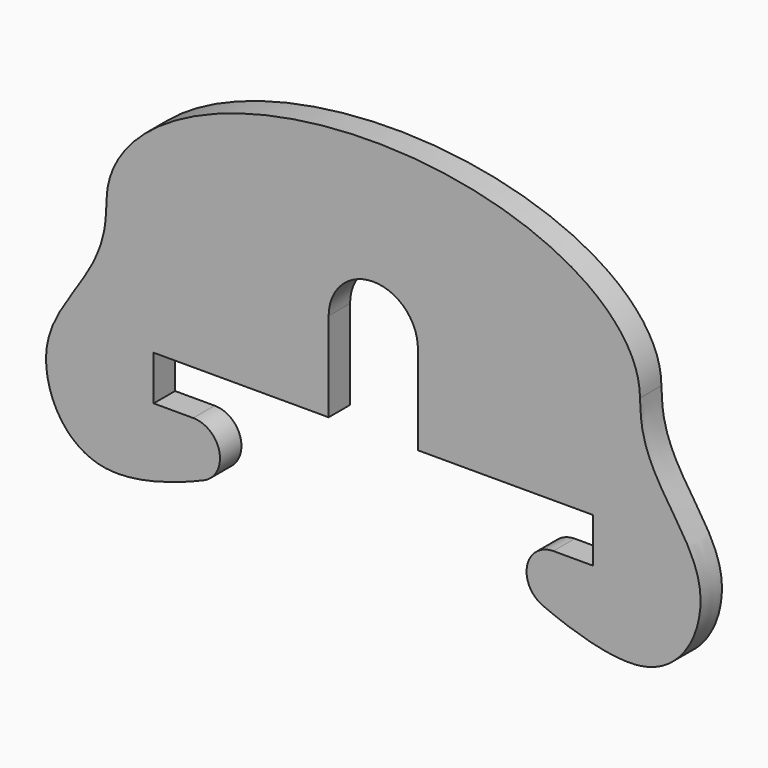
from build123d import *

# Parameters (mm, degrees)
F1_DEPTH = 3


# Not quite as in the source:
# - ends of sketch curves that miss each other by under 0.0002 mm in the source are joined
# - the dataset's text gives a spline's control points without its knots; the knots are read off the source's solid


with BuildPart() as f1:
    # F0 (on Front) → F1 (new body)
    with BuildSketch(Plane.XZ):
        with BuildLine():
            Line((-20.166137, -12.809077), (-24.6, -12.809077))
            Line((-24.6, -12.809077), (-24.6, -7.809077))
            Line((-24.6, -7.809077), (-5, -7.809077))
            Line((-5, -7.809077), (-5, 2.190923))
            ThreePointArc((-5, 2.190923), (0, 7.190923), (5, 2.190923))
            Line((5, 2.190923), (5, -7.809077))
            Line((5, -7.809077), (24.6, -7.809077))
            Line((24.6, -7.809077), (24.6, -12.809077))
            Line((24.6, -12.809077), (20.166138, -12.809077))
            ThreePointArc((20.166138, -12.809077), (17.2280963794, -15.2025199657), (18.9780781253, -18.5638027094))
            add(Edge.make_bspline(
                [(29.869969, 5.432538), (29.917769, 4.949314), (29.942006, -2.148841), (40.01044, -8.831034), (33.118633, -23.880184), (21.728451, -19.749985), (18.9780781253, -18.5638027094)],
                knots=[26.688985, 26.688985, 26.688985, 26.688985, 28.557776, 42.872008, 54.1154, 62.665306, 62.665306, 62.665306, 62.665306], degree=3))
            add(Edge.make_bspline(
                [(29.869969, 5.432538), (29.869969, 21.0209257), (-5.1736e-06, 21.020923), (-29.8699793473, 21.0209203), (-29.869969, 5.4325326)],
                knots=[0, 0, 0, 1.5707965, 1.5707965, 3.141593, 3.141593, 3.141593], degree=2, weights=[1, 0.7071067199, 1, 0.7071067199, 1]))
            add(Edge.make_bspline(
                [(-29.869969, 5.4325326), (-29.917769, 4.949314), (-29.942006, -2.148841), (-40.01044, -8.831034), (-33.118633, -23.880184), (-21.72845, -19.749985), (-18.978078, -18.563803)],
                knots=[26.688985, 26.688985, 26.688985, 26.688985, 28.557776, 42.872008, 54.1154, 62.665306, 62.665306, 62.665306, 62.665306], degree=3))
            ThreePointArc((-18.978078, -18.563803), (-17.2280952866, -15.2025204153), (-20.166137, -12.809077))
        make_face()
    extrude(amount=F1_DEPTH)


solid = f1.part
